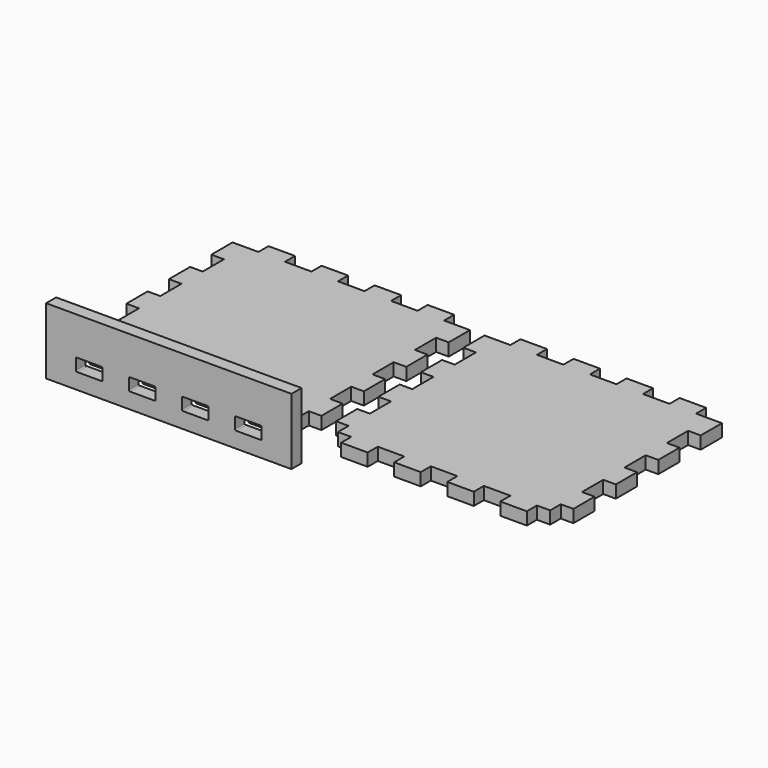
from build123d import *

# Parameters (mm, degrees)
F1_W          = 19
F1_H          = 40
F1_W_2        = 40
F1_H_2        = 19
F2_DEPTH      = 19
F4_W          = 370
F4_H          = 100
F5_DEPTH      = 19
F6_DEPTH      = 188
F7_R          = 1.5
F8_T1_DEPTH   = 17.5
F8_T6_ANGLE   = 233.3892475384
F8_T11_ANGLE  = 233.3892475384
F8_T16_ANGLE  = 233.3892475384
F8_T21_ANGLE  = 233.3892475384
F8_T26_ANGLE  = 233.3892475384
F8_T31_ANGLE  = 233.3892475384
F8_T36_ANGLE  = 233.3892475384
F8_T41_ANGLE  = 233.3892475384
F8_T46_ANGLE  = 233.3892475384
F8_T51_ANGLE  = 233.3892475384
F8_T56_ANGLE  = 233.3892475384
F8_T61_ANGLE  = 233.3892475384
F8_T66_ANGLE  = 233.3892475384
F8_T71_ANGLE  = 233.3892475384
F8_T76_ANGLE  = 233.3892475384
F8_T81_ANGLE  = 233.3892475384
F9_R          = 1.5
F10_T1_DEPTH  = 16
F10_T6_ANGLE  = 233.2969892374
F10_T11_ANGLE = 233.2969892374
F10_T16_ANGLE = 233.2969892374
F10_T21_ANGLE = 233.2969892374
F10_T26_ANGLE = 233.2969892374
F10_T31_ANGLE = 233.2969892374
F10_T36_ANGLE = 233.2969892374
F10_T41_ANGLE = 233.2969892374
F10_T46_ANGLE = 233.2969892374
F10_T51_ANGLE = 233.2969892374
F10_T56_ANGLE = 233.2969892374
F10_T61_ANGLE = 233.2969892374
F10_T66_ANGLE = 233.2969892374
F10_T71_ANGLE = 233.2969892374
F10_T76_ANGLE = 233.2969892374
F10_T81_ANGLE = 233.2969892374
F11_R         = 2.5
F12_DEPTH     = 1


# Not quite as in the source:
# - a fillet or chamfer that OpenCascade refuses, or shapes differently, is made with other operations: its cross-section is extruded or revolved along the edge and cut away or added


with BuildPart() as f2:
    # F1 (on Top) → F2 (new body)
    with BuildSketch(Plane.XY):
        with Locations((15.5, 65)):
            Rectangle(F1_W, F1_H)
        with Locations((15.5, 145)):
            Rectangle(F1_W, F1_H)
        Polygon((25, 85), (25, 45), (25, 25), (45, 25), (85, 25), (125, 25), (165, 25), (205, 25), (245, 25), (285, 25), (325, 25), (345, 25), (345, 45), (345, 85), (345, 125), (345, 165), (345, 205), (345, 245), (345, 285), (345, 325), (325, 325), (285, 325), (245, 325), (205, 325), (165, 325), (125, 325), (85, 325), (45, 325), (25, 325), (25, 285), (25, 245), (25, 205), (25, 165), (25, 125), align=None)
        with Locations((354.5, 65)):
            Rectangle(F1_W, F1_H)
        with Locations((305, 334.5)):
            Rectangle(F1_W_2, F1_H_2)
        with Locations((15.5, 225)):
            Rectangle(F1_W, F1_H)
        with Locations((15.5, 305)):
            Rectangle(F1_W, F1_H)
        with Locations((354.5, 225)):
            Rectangle(F1_W, F1_H)
        with Locations((354.5, 145)):
            Rectangle(F1_W, F1_H)
        with Locations((305, 15.5)):
            Rectangle(F1_W_2, F1_H_2)
        with Locations((225, 15.5)):
            Rectangle(F1_W_2, F1_H_2)
        with Locations((145, 334.5)):
            Rectangle(F1_W_2, F1_H_2)
        with Locations((225, 334.5)):
            Rectangle(F1_W_2, F1_H_2)
        with Locations((145, 15.5)):
            Rectangle(F1_W_2, F1_H_2)
        with Locations((65, 15.5)):
            Rectangle(F1_W_2, F1_H_2)
        with Locations((65, 334.5)):
            Rectangle(F1_W_2, F1_H_2)
        with Locations((354.5, 305)):
            Rectangle(F1_W, F1_H)
    extrude(amount=F2_DEPTH)


with BuildPart() as f3_1:
    # F3: copy of F2
    add(f2.part.moved(Location((380, 0, 0))))


with BuildPart() as f5:
    # F4 (on Front) → F5 (new body)
    with BuildSketch(Plane.XZ):
        with Locations((185, 26.175237447)):
            Rectangle(F4_W, F4_H)
    extrude(amount=F5_DEPTH)

    # F6 (cut): faces of the model
    f6_faces = [f2.part.faces().sort_by_distance(p)[0] for p in [
        (65, 6, 9.5),
        (145, 6, 9.5),
        (225, 6, 9.5),
        (305, 6, 9.5),
    ]]
    extrude(f6_faces, amount=F6_DEPTH, mode=Mode.SUBTRACT)

    # F7
    f7_edges = [f5.edges().sort_by_distance(p)[0] for p in [
        (325, 0, 9.5),
        (285, 0, 9.5),
        (245, 0, 9.5),
        (205, 0, 9.5),
        (165, 0, 9.5),
        (125, 0, 9.5),
        (85, 0, 9.5),
        (45, 0, 9.5),
    ]]
    fillet(f7_edges, radius=F7_R)

    # F8: fillet of radius 1.5 on 16 edges, made by hand

    # F8_s2 → F8_t1 (join)
    with BuildSketch(Plane.XZ.offset(1.5)):
        with BuildLine():
            ThreePointArc((46.5009656854, 19.0004), (45.4393398282, 18.5606601718), (44.9996, 17.4990343146))
            Line((44.9996, 17.4990343146), (44.8494634315, 17.4990343146))
            ThreePointArc((44.8494634315, 17.4990343146), (44.8498634315, 18.2495171573), (44.8498634315, 19))
            Line((44.8498634315, 19), (45, 19.1501365685))
            ThreePointArc((45, 19.1501365685), (45.7504828427, 19.1501365685), (46.5009656854, 19.1505365685))
            Line((46.5009656854, 19.1505365685), (46.5009656854, 19.0004))
        make_face()
        with BuildLine():
            ThreePointArc((46.5009656854, -0.0004), (45.4393398282, 0.4393398282), (44.9996, 1.5009656854))
            Line((44.9996, 1.5009656854), (44.8494634315, 1.5009656854))
            ThreePointArc((44.8494634315, 1.5009656854), (44.8498634315, 0.7504828427), (44.8498634315, 0))
            Line((44.8498634315, 0), (45, -0.1501365685))
            ThreePointArc((45, -0.1501365685), (45.7504828427, -0.1501365685), (46.5009656854, -0.1505365685))
            Line((46.5009656854, -0.1505365685), (46.5009656854, -0.0004))
        make_face()
        with BuildLine():
            ThreePointArc((83.4990343146, 19.0004), (84.5606601718, 18.5606601718), (85.0004, 17.4990343146))
            Line((85.0004, 17.4990343146), (85.1505365685, 17.4990343146))
            ThreePointArc((85.1505365685, 17.4990343146), (85.1501365685, 18.2495171573), (85.1501365685, 19))
            Line((85.1501365685, 19), (85, 19.1501365685))
            ThreePointArc((85, 19.1501365685), (84.2495171573, 19.1501365685), (83.4990343146, 19.1505365685))
            Line((83.4990343146, 19.1505365685), (83.4990343146, 19.0004))
        make_face()
        with BuildLine():
            ThreePointArc((83.4990343146, -0.0004), (84.5606601718, 0.4393398282), (85.0004, 1.5009656854))
            Line((85.0004, 1.5009656854), (85.1505365685, 1.5009656854))
            ThreePointArc((85.1505365685, 1.5009656854), (85.1501365685, 0.7504828427), (85.1501365685, 0))
            Line((85.1501365685, 0), (85, -0.1501365685))
            ThreePointArc((85, -0.1501365685), (84.2495171573, -0.1501365685), (83.4990343146, -0.1505365685))
            Line((83.4990343146, -0.1505365685), (83.4990343146, -0.0004))
        make_face()
        with BuildLine():
            ThreePointArc((126.5009656854, 19.0004), (125.4393398282, 18.5606601718), (124.9996, 17.4990343146))
            Line((124.9996, 17.4990343146), (124.8494634315, 17.4990343146))
            ThreePointArc((124.8494634315, 17.4990343146), (124.8498634315, 18.2495171573), (124.8498634315, 19))
            Line((124.8498634315, 19), (125, 19.1501365685))
            ThreePointArc((125, 19.1501365685), (125.7504828427, 19.1501365685), (126.5009656854, 19.1505365685))
            Line((126.5009656854, 19.1505365685), (126.5009656854, 19.0004))
        make_face()
        with BuildLine():
            ThreePointArc((126.5009656854, -0.0004), (125.4393398282, 0.4393398282), (124.9996, 1.5009656854))
            Line((124.9996, 1.5009656854), (124.8494634315, 1.5009656854))
            ThreePointArc((124.8494634315, 1.5009656854), (124.8498634315, 0.7504828427), (124.8498634315, 0))
            Line((124.8498634315, 0), (125, -0.1501365685))
            ThreePointArc((125, -0.1501365685), (125.7504828427, -0.1501365685), (126.5009656854, -0.1505365685))
            Line((126.5009656854, -0.1505365685), (126.5009656854, -0.0004))
        make_face()
        with BuildLine():
            ThreePointArc((163.4990343146, -0.0004), (164.5606601718, 0.4393398282), (165.0004, 1.5009656854))
            Line((165.0004, 1.5009656854), (165.1505365685, 1.5009656854))
            ThreePointArc((165.1505365685, 1.5009656854), (165.1501365685, 0.7504828427), (165.1501365685, 0))
            Line((165.1501365685, 0), (165, -0.1501365685))
            ThreePointArc((165, -0.1501365685), (164.2495171573, -0.1501365685), (163.4990343146, -0.1505365685))
            Line((163.4990343146, -0.1505365685), (163.4990343146, -0.0004))
        make_face()
        with BuildLine():
            ThreePointArc((206.5009656854, -0.0004), (205.4393398282, 0.4393398282), (204.9996, 1.5009656854))
            Line((204.9996, 1.5009656854), (204.8494634315, 1.5009656854))
            ThreePointArc((204.8494634315, 1.5009656854), (204.8498634315, 0.7504828427), (204.8498634315, 0))
            Line((204.8498634315, 0), (205, -0.1501365685))
            ThreePointArc((205, -0.1501365685), (205.7504828427, -0.1501365685), (206.5009656854, -0.1505365685))
            Line((206.5009656854, -0.1505365685), (206.5009656854, -0.0004))
        make_face()
        with BuildLine():
            ThreePointArc((206.5009656854, 19.0004), (205.4393398282, 18.5606601718), (204.9996, 17.4990343146))
            Line((204.9996, 17.4990343146), (204.8494634315, 17.4990343146))
            ThreePointArc((204.8494634315, 17.4990343146), (204.8498634315, 18.2495171573), (204.8498634315, 19))
            Line((204.8498634315, 19), (205, 19.1501365685))
            ThreePointArc((205, 19.1501365685), (205.7504828427, 19.1501365685), (206.5009656854, 19.1505365685))
            Line((206.5009656854, 19.1505365685), (206.5009656854, 19.0004))
        make_face()
        with BuildLine():
            ThreePointArc((243.4990343146, -0.0004), (244.5606601718, 0.4393398282), (245.0004, 1.5009656854))
            Line((245.0004, 1.5009656854), (245.1505365685, 1.5009656854))
            ThreePointArc((245.1505365685, 1.5009656854), (245.1501365685, 0.7504828427), (245.1501365685, 0))
            Line((245.1501365685, 0), (245, -0.1501365685))
            ThreePointArc((245, -0.1501365685), (244.2495171573, -0.1501365685), (243.4990343146, -0.1505365685))
            Line((243.4990343146, -0.1505365685), (243.4990343146, -0.0004))
        make_face()
        with BuildLine():
            ThreePointArc((243.4990343146, 19.0004), (244.5606601718, 18.5606601718), (245.0004, 17.4990343146))
            Line((245.0004, 17.4990343146), (245.1505365685, 17.4990343146))
            ThreePointArc((245.1505365685, 17.4990343146), (245.1501365685, 18.2495171573), (245.1501365685, 19))
            Line((245.1501365685, 19), (245, 19.1501365685))
            ThreePointArc((245, 19.1501365685), (244.2495171573, 19.1501365685), (243.4990343146, 19.1505365685))
            Line((243.4990343146, 19.1505365685), (243.4990343146, 19.0004))
        make_face()
        with BuildLine():
            ThreePointArc((323.4990343146, 19.0004), (324.5606601718, 18.5606601718), (325.0004, 17.4990343146))
            Line((325.0004, 17.4990343146), (325.1505365685, 17.4990343146))
            ThreePointArc((325.1505365685, 17.4990343146), (325.1501365685, 18.2495171573), (325.1501365685, 19))
            Line((325.1501365685, 19), (325, 19.1501365685))
            ThreePointArc((325, 19.1501365685), (324.2495171573, 19.1501365685), (323.4990343146, 19.1505365685))
            Line((323.4990343146, 19.1505365685), (323.4990343146, 19.0004))
        make_face()
        with BuildLine():
            ThreePointArc((286.5009656854, 19.0004), (285.4393398282, 18.5606601718), (284.9996, 17.4990343146))
            Line((284.9996, 17.4990343146), (284.8494634315, 17.4990343146))
            ThreePointArc((284.8494634315, 17.4990343146), (284.8498634315, 18.2495171573), (284.8498634315, 19))
            Line((284.8498634315, 19), (285, 19.1501365685))
            ThreePointArc((285, 19.1501365685), (285.7504828427, 19.1501365685), (286.5009656854, 19.1505365685))
            Line((286.5009656854, 19.1505365685), (286.5009656854, 19.0004))
        make_face()
        with BuildLine():
            ThreePointArc((163.4990343146, 19.0004), (164.5606601718, 18.5606601718), (165.0004, 17.4990343146))
            Line((165.0004, 17.4990343146), (165.1505365685, 17.4990343146))
            ThreePointArc((165.1505365685, 17.4990343146), (165.1501365685, 18.2495171573), (165.1501365685, 19))
            Line((165.1501365685, 19), (165, 19.1501365685))
            ThreePointArc((165, 19.1501365685), (164.2495171573, 19.1501365685), (163.4990343146, 19.1505365685))
            Line((163.4990343146, 19.1505365685), (163.4990343146, 19.0004))
        make_face()
        with BuildLine():
            ThreePointArc((286.5009656854, -0.0004), (285.4393398282, 0.4393398282), (284.9996, 1.5009656854))
            Line((284.9996, 1.5009656854), (284.8494634315, 1.5009656854))
            ThreePointArc((284.8494634315, 1.5009656854), (284.8498634315, 0.7504828427), (284.8498634315, 0))
            Line((284.8498634315, 0), (285, -0.1501365685))
            ThreePointArc((285, -0.1501365685), (285.7504828427, -0.1501365685), (286.5009656854, -0.1505365685))
            Line((286.5009656854, -0.1505365685), (286.5009656854, -0.0004))
        make_face()
        with BuildLine():
            ThreePointArc((323.4990343146, -0.0004), (324.5606601718, 0.4393398282), (325.0004, 1.5009656854))
            Line((325.0004, 1.5009656854), (325.1505365685, 1.5009656854))
            ThreePointArc((325.1505365685, 1.5009656854), (325.1501365685, 0.7504828427), (325.1501365685, 0))
            Line((325.1501365685, 0), (325, -0.1501365685))
            ThreePointArc((325, -0.1501365685), (324.2495171573, -0.1501365685), (323.4990343146, -0.1505365685))
            Line((323.4990343146, -0.1505365685), (323.4990343146, -0.0004))
        make_face()
    extrude(amount=F8_T1_DEPTH)


with BuildPart() as f8_tool4:
    # F8_s5 → F8_t6 (revolve)
    with BuildSketch(Plane(origin=(209.6577088502, 155.7666111289, 0), x_dir=(0, 0, 1), z_dir=(-0.80270557, -0.5963755259, 0))):
        with BuildLine():
            ThreePointArc((1.5009656854, -197.4202675598), (0.4393398282, -197.8600073881), (-0.0004, -198.9216332453))
            Line((-0.0004, -198.9216332453), (-0.1505365685, -198.9216332453))
            ThreePointArc((-0.1505365685, -198.9216332453), (-0.1501365685, -198.1711504026), (-0.1501365685, -197.4206675598))
            Line((-0.1501365685, -197.4206675598), (0, -197.2705309913))
            ThreePointArc((0, -197.2705309913), (0.7504828427, -197.2705309913), (1.5009656854, -197.2701309913))
            Line((1.5009656854, -197.2701309913), (1.5009656854, -197.4202675598))
        make_face()
    revolve(axis=Axis((326.5, -1.5, 0), (0, 0, 1)), revolution_arc=F8_T6_ANGLE)

    split(bisect_by=Plane.XZ, keep=Keep.TOP)


with BuildPart() as f5_1:
    add(f5.part)

    # F8_t3: union F8_tool4
    add(f8_tool4.part)


with BuildPart() as f8_tool9:
    # F8_s10 → F8_t11 (revolve)
    with BuildSketch(Plane(origin=(183.3873927387, -136.2489023052, 0), x_dir=(0, 0, 1), z_dir=(0.80270557, -0.5963755259, 0))):
        with BuildLine():
            ThreePointArc((-0.0004, -164.8674375509), (0.4393398282, -165.9290634081), (1.5009656854, -166.3688032363))
            Line((1.5009656854, -166.3688032363), (1.5009656854, -166.5189398049))
            ThreePointArc((1.5009656854, -166.5189398049), (0.7504828427, -166.5185398049), (0, -166.5185398049))
            Line((0, -166.5185398049), (-0.1501365685, -166.3684032363))
            ThreePointArc((-0.1501365685, -166.3684032363), (-0.1501365685, -165.6179203936), (-0.1505365685, -164.8674375509))
            Line((-0.1505365685, -164.8674375509), (-0.0004, -164.8674375509))
        make_face()
    revolve(axis=Axis((283.5, -1.5, 0), (0, 0, -1)), revolution_arc=F8_T11_ANGLE)

    split(bisect_by=Plane.XZ, keep=Keep.TOP)


with BuildPart() as f5_2:
    add(f5_1.part)

    # F8_t8: union F8_tool9
    add(f8_tool9.part)


with BuildPart() as f8_tool14:
    # F8_s15 → F8_t16 (revolve)
    with BuildSketch(Plane(origin=(106.5639117121, 79.172378097, 0), x_dir=(0, 0, 1), z_dir=(-0.80270557, -0.5963755259, 0))):
        with BuildLine():
            ThreePointArc((19.0004, -103.501549102), (18.5606601718, -102.4399232448), (17.4990343146, -102.0001834166))
            Line((17.4990343146, -102.0001834166), (17.4990343146, -101.850046848))
            ThreePointArc((17.4990343146, -101.850046848), (18.2495171573, -101.850446848), (19, -101.850446848))
            Line((19, -101.850446848), (19.1501365685, -102.0005834166))
            ThreePointArc((19.1501365685, -102.0005834166), (19.1501365685, -102.7510662593), (19.1505365685, -103.501549102))
            Line((19.1505365685, -103.501549102), (19.0004, -103.501549102))
        make_face()
    revolve(axis=Axis((166.5, -1.5, 19), (0, 0, 1)), revolution_arc=F8_T16_ANGLE)

    split(bisect_by=Plane.XZ, keep=Keep.TOP)


with BuildPart() as f5_3:
    add(f5_2.part)

    # F8_t13: union F8_tool14
    add(f8_tool14.part)


with BuildPart() as f8_tool19:
    # F8_s20 → F8_t21 (revolve)
    with BuildSketch(Plane(origin=(183.3873927387, -136.2489023052, 0), x_dir=(0, 0, 1), z_dir=(0.80270557, -0.5963755259, 0))):
        with BuildLine():
            ThreePointArc((19.0004, -164.8674375509), (18.5606601718, -165.9290634081), (17.4990343146, -166.3688032363))
            Line((17.4990343146, -166.3688032363), (17.4990343146, -166.5189398049))
            ThreePointArc((17.4990343146, -166.5189398049), (18.2495171573, -166.5185398049), (19, -166.5185398049))
            Line((19, -166.5185398049), (19.1501365685, -166.3684032363))
            ThreePointArc((19.1501365685, -166.3684032363), (19.1501365685, -165.6179203936), (19.1505365685, -164.8674375509))
            Line((19.1505365685, -164.8674375509), (19.0004, -164.8674375509))
        make_face()
    revolve(axis=Axis((283.5, -1.5, 19), (0, 0, -1)), revolution_arc=F8_T21_ANGLE)

    split(bisect_by=Plane.XZ, keep=Keep.TOP)


with BuildPart() as f5_4:
    add(f5_3.part)

    # F8_t18: union F8_tool19
    add(f8_tool19.part)


with BuildPart() as f8_tool24:
    # F8_s25 → F8_t26 (revolve)
    with BuildSketch(Plane(origin=(209.6577088502, 155.7666111289, 0), x_dir=(0, 0, 1), z_dir=(-0.80270557, -0.5963755259, 0))):
        with BuildLine():
            ThreePointArc((19.0004, -198.9216332453), (18.5606601718, -197.8600073881), (17.4990343146, -197.4202675598))
            Line((17.4990343146, -197.4202675598), (17.4990343146, -197.2701309913))
            ThreePointArc((17.4990343146, -197.2701309913), (18.2495171573, -197.2705309913), (19, -197.2705309913))
            Line((19, -197.2705309913), (19.1501365685, -197.4206675598))
            ThreePointArc((19.1501365685, -197.4206675598), (19.1501365685, -198.1711504026), (19.1505365685, -198.9216332453))
            Line((19.1505365685, -198.9216332453), (19.0004, -198.9216332453))
        make_face()
    revolve(axis=Axis((326.5, -1.5, 19), (0, 0, 1)), revolution_arc=F8_T26_ANGLE)

    split(bisect_by=Plane.XZ, keep=Keep.TOP)


with BuildPart() as f5_5:
    add(f5_4.part)

    # F8_t23: union F8_tool24
    add(f8_tool24.part)


with BuildPart() as f8_tool29:
    # F8_s30 → F8_t31 (revolve)
    with BuildSketch(Plane(origin=(158.1108102812, 117.4694946129, 0), x_dir=(0, 0, 1), z_dir=(-0.80270557, -0.5963755259, 0))):
        with BuildLine():
            ThreePointArc((19.0004, -151.2115911736), (18.5606601718, -150.1499653164), (17.4990343146, -149.7102254882))
            Line((17.4990343146, -149.7102254882), (17.4990343146, -149.5600889197))
            ThreePointArc((17.4990343146, -149.5600889197), (18.2495171573, -149.5604889197), (19, -149.5604889197))
            Line((19, -149.5604889197), (19.1501365685, -149.7106254882))
            ThreePointArc((19.1501365685, -149.7106254882), (19.1501365685, -150.4611083309), (19.1505365685, -151.2115911736))
            Line((19.1505365685, -151.2115911736), (19.0004, -151.2115911736))
        make_face()
    revolve(axis=Axis((246.5, -1.5, 19), (0, 0, 1)), revolution_arc=F8_T31_ANGLE)

    split(bisect_by=Plane.XZ, keep=Keep.TOP)


with BuildPart() as f5_6:
    add(f5_5.part)

    # F8_t28: union F8_tool29
    add(f8_tool29.part)


with BuildPart() as f8_tool34:
    # F8_s35 → F8_t36 (revolve)
    with BuildSketch(Plane(origin=(158.1108102812, 117.4694946129, 0), x_dir=(0, 0, 1), z_dir=(-0.80270557, -0.5963755259, 0))):
        with BuildLine():
            ThreePointArc((1.5009656854, -149.7102254882), (0.4393398282, -150.1499653164), (-0.0004, -151.2115911736))
            Line((-0.0004, -151.2115911736), (-0.1505365685, -151.2115911736))
            ThreePointArc((-0.1505365685, -151.2115911736), (-0.1501365685, -150.4611083309), (-0.1501365685, -149.7106254882))
            Line((-0.1501365685, -149.7106254882), (0, -149.5604889197))
            ThreePointArc((0, -149.5604889197), (0.7504828427, -149.5604889197), (1.5009656854, -149.5600889197))
            Line((1.5009656854, -149.5600889197), (1.5009656854, -149.7102254882))
        make_face()
    revolve(axis=Axis((246.5, -1.5, 0), (0, 0, 1)), revolution_arc=F8_T36_ANGLE)

    split(bisect_by=Plane.XZ, keep=Keep.TOP)


with BuildPart() as f5_7:
    add(f5_6.part)

    # F8_t33: union F8_tool34
    add(f8_tool34.part)


with BuildPart() as f8_tool39:
    # F8_s40 → F8_t41 (revolve)
    with BuildSketch(Plane(origin=(131.8404941697, -97.9517857893, 0), x_dir=(0, 0, 1), z_dir=(0.80270557, -0.5963755259, 0))):
        with BuildLine():
            ThreePointArc((19.0004, -117.1573954793), (18.5606601718, -118.2190213365), (17.4990343146, -118.6587611647))
            Line((17.4990343146, -118.6587611647), (17.4990343146, -118.8088977333))
            ThreePointArc((17.4990343146, -118.8088977333), (18.2495171573, -118.8084977333), (19, -118.8084977333))
            Line((19, -118.8084977333), (19.1501365685, -118.6583611647))
            ThreePointArc((19.1501365685, -118.6583611647), (19.1501365685, -117.907878322), (19.1505365685, -117.1573954793))
            Line((19.1505365685, -117.1573954793), (19.0004, -117.1573954793))
        make_face()
    revolve(axis=Axis((203.5, -1.5, 19), (0, 0, -1)), revolution_arc=F8_T41_ANGLE)

    split(bisect_by=Plane.XZ, keep=Keep.TOP)


with BuildPart() as f5_8:
    add(f5_7.part)

    # F8_t38: union F8_tool39
    add(f8_tool39.part)


with BuildPart() as f8_tool44:
    # F8_s45 → F8_t46 (revolve)
    with BuildSketch(Plane(origin=(131.8404941697, -97.9517857893, 0), x_dir=(0, 0, 1), z_dir=(0.80270557, -0.5963755259, 0))):
        with BuildLine():
            ThreePointArc((-0.0004, -117.1573954793), (0.4393398282, -118.2190213365), (1.5009656854, -118.6587611647))
            Line((1.5009656854, -118.6587611647), (1.5009656854, -118.8088977333))
            ThreePointArc((1.5009656854, -118.8088977333), (0.7504828427, -118.8084977333), (0, -118.8084977333))
            Line((0, -118.8084977333), (-0.1501365685, -118.6583611647))
            ThreePointArc((-0.1501365685, -118.6583611647), (-0.1501365685, -117.907878322), (-0.1505365685, -117.1573954793))
            Line((-0.1505365685, -117.1573954793), (-0.0004, -117.1573954793))
        make_face()
    revolve(axis=Axis((203.5, -1.5, 0), (0, 0, -1)), revolution_arc=F8_T46_ANGLE)

    split(bisect_by=Plane.XZ, keep=Keep.TOP)


with BuildPart() as f5_9:
    add(f5_8.part)

    # F8_t43: union F8_tool44
    add(f8_tool44.part)


with BuildPart() as f8_tool49:
    # F8_s50 → F8_t51 (revolve)
    with BuildSketch(Plane(origin=(106.5639117121, 79.172378097, 0), x_dir=(0, 0, 1), z_dir=(-0.80270557, -0.5963755259, 0))):
        with BuildLine():
            ThreePointArc((1.5009656854, -102.0001834166), (0.4393398282, -102.4399232448), (-0.0004, -103.501549102))
            Line((-0.0004, -103.501549102), (-0.1505365685, -103.501549102))
            ThreePointArc((-0.1505365685, -103.501549102), (-0.1501365685, -102.7510662593), (-0.1501365685, -102.0005834166))
            Line((-0.1501365685, -102.0005834166), (0, -101.850446848))
            ThreePointArc((0, -101.850446848), (0.7504828427, -101.850446848), (1.5009656854, -101.850046848))
            Line((1.5009656854, -101.850046848), (1.5009656854, -102.0001834166))
        make_face()
    revolve(axis=Axis((166.5, -1.5, 0), (0, 0, 1)), revolution_arc=F8_T51_ANGLE)

    split(bisect_by=Plane.XZ, keep=Keep.TOP)


with BuildPart() as f5_10:
    add(f5_9.part)

    # F8_t48: union F8_tool49
    add(f8_tool49.part)


with BuildPart() as f8_tool54:
    # F8_s55 → F8_t56 (revolve)
    with BuildSketch(Plane(origin=(80.2935956006, -59.6546692733, 0), x_dir=(0, 0, 1), z_dir=(0.80270557, -0.5963755259, 0))):
        with BuildLine():
            ThreePointArc((-0.0004, -69.4473534077), (0.4393398282, -70.5089792649), (1.5009656854, -70.9487190931))
            Line((1.5009656854, -70.9487190931), (1.5009656854, -71.0988556616))
            ThreePointArc((1.5009656854, -71.0988556616), (0.7504828427, -71.0984556616), (0, -71.0984556616))
            Line((0, -71.0984556616), (-0.1501365685, -70.9483190931))
            ThreePointArc((-0.1501365685, -70.9483190931), (-0.1501365685, -70.1978362504), (-0.1505365685, -69.4473534077))
            Line((-0.1505365685, -69.4473534077), (-0.0004, -69.4473534077))
        make_face()
    revolve(axis=Axis((123.5, -1.5, 0), (0, 0, -1)), revolution_arc=F8_T56_ANGLE)

    split(bisect_by=Plane.XZ, keep=Keep.TOP)


with BuildPart() as f5_11:
    add(f5_10.part)

    # F8_t53: union F8_tool54
    add(f8_tool54.part)


with BuildPart() as f8_tool59:
    # F8_s60 → F8_t61 (revolve)
    with BuildSketch(Plane(origin=(80.2935956006, -59.6546692733, 0), x_dir=(0, 0, 1), z_dir=(0.80270557, -0.5963755259, 0))):
        with BuildLine():
            ThreePointArc((19.0004, -69.4473534077), (18.5606601718, -70.5089792649), (17.4990343146, -70.9487190931))
            Line((17.4990343146, -70.9487190931), (17.4990343146, -71.0988556616))
            ThreePointArc((17.4990343146, -71.0988556616), (18.2495171573, -71.0984556616), (19, -71.0984556616))
            Line((19, -71.0984556616), (19.1501365685, -70.9483190931))
            ThreePointArc((19.1501365685, -70.9483190931), (19.1501365685, -70.1978362504), (19.1505365685, -69.4473534077))
            Line((19.1505365685, -69.4473534077), (19.0004, -69.4473534077))
        make_face()
    revolve(axis=Axis((123.5, -1.5, 19), (0, 0, -1)), revolution_arc=F8_T61_ANGLE)

    split(bisect_by=Plane.XZ, keep=Keep.TOP)


with BuildPart() as f5_12:
    add(f5_11.part)

    # F8_t58: union F8_tool59
    add(f8_tool59.part)


with BuildPart() as f8_tool64:
    # F8_s65 → F8_t66 (revolve)
    with BuildSketch(Plane(origin=(55.0170131431, 40.875261581, 0), x_dir=(0, 0, 1), z_dir=(-0.80270557, -0.5963755259, 0))):
        with BuildLine():
            ThreePointArc((1.5009656854, -54.290141345), (0.4393398282, -54.7298811732), (-0.0004, -55.7915070304))
            Line((-0.0004, -55.7915070304), (-0.1505365685, -55.7915070304))
            ThreePointArc((-0.1505365685, -55.7915070304), (-0.1501365685, -55.0410241877), (-0.1501365685, -54.290541345))
            Line((-0.1501365685, -54.290541345), (0, -54.1404047764))
            ThreePointArc((0, -54.1404047764), (0.7504828427, -54.1404047764), (1.5009656854, -54.1400047764))
            Line((1.5009656854, -54.1400047764), (1.5009656854, -54.290141345))
        make_face()
    revolve(axis=Axis((86.5, -1.5, 0), (0, 0, 1)), revolution_arc=F8_T66_ANGLE)

    split(bisect_by=Plane.XZ, keep=Keep.TOP)


with BuildPart() as f5_13:
    add(f5_12.part)

    # F8_t63: union F8_tool64
    add(f8_tool64.part)


with BuildPart() as f8_tool69:
    # F8_s70 → F8_t71 (revolve)
    with BuildSketch(Plane(origin=(55.0170131431, 40.875261581, 0), x_dir=(0, 0, 1), z_dir=(-0.80270557, -0.5963755259, 0))):
        with BuildLine():
            ThreePointArc((19.0004, -55.7915070304), (18.5606601718, -54.7298811732), (17.4990343146, -54.290141345))
            Line((17.4990343146, -54.290141345), (17.4990343146, -54.1400047764))
            ThreePointArc((17.4990343146, -54.1400047764), (18.2495171573, -54.1404047764), (19, -54.1404047764))
            Line((19, -54.1404047764), (19.1501365685, -54.290541345))
            ThreePointArc((19.1501365685, -54.290541345), (19.1501365685, -55.0410241877), (19.1505365685, -55.7915070304))
            Line((19.1505365685, -55.7915070304), (19.0004, -55.7915070304))
        make_face()
    revolve(axis=Axis((86.5, -1.5, 19), (0, 0, 1)), revolution_arc=F8_T71_ANGLE)

    split(bisect_by=Plane.XZ, keep=Keep.TOP)


with BuildPart() as f5_14:
    add(f5_13.part)

    # F8_t68: union F8_tool69
    add(f8_tool69.part)


with BuildPart() as f8_tool74:
    # F8_s75 → F8_t76 (revolve)
    with BuildSketch(Plane(origin=(28.7466970316, -21.3575527574, 0), x_dir=(0, 0, 1), z_dir=(0.80270557, -0.5963755259, 0))):
        with BuildLine():
            ThreePointArc((-0.0004, -21.737311336), (0.4393398282, -22.7989371932), (1.5009656854, -23.2386770214))
            Line((1.5009656854, -23.2386770214), (1.5009656854, -23.38881359))
            ThreePointArc((1.5009656854, -23.38881359), (0.7504828427, -23.38841359), (0, -23.38841359))
            Line((0, -23.38841359), (-0.1501365685, -23.2382770214))
            ThreePointArc((-0.1501365685, -23.2382770214), (-0.1501365685, -22.4877941787), (-0.1505365685, -21.737311336))
            Line((-0.1505365685, -21.737311336), (-0.0004, -21.737311336))
        make_face()
    revolve(axis=Axis((43.5, -1.5, 0), (0, 0, -1)), revolution_arc=F8_T76_ANGLE)

    split(bisect_by=Plane.XZ, keep=Keep.TOP)


with BuildPart() as f5_15:
    add(f5_14.part)

    # F8_t73: union F8_tool74
    add(f8_tool74.part)


with BuildPart() as f8_tool79:
    # F8_s80 → F8_t81 (revolve)
    with BuildSketch(Plane(origin=(28.7466970316, -21.3575527574, 0), x_dir=(0, 0, 1), z_dir=(0.80270557, -0.5963755259, 0))):
        with BuildLine():
            ThreePointArc((19.0004, -21.737311336), (18.5606601718, -22.7989371932), (17.4990343146, -23.2386770214))
            Line((17.4990343146, -23.2386770214), (17.4990343146, -23.38881359))
            ThreePointArc((17.4990343146, -23.38881359), (18.2495171573, -23.38841359), (19, -23.38841359))
            Line((19, -23.38841359), (19.1501365685, -23.2382770214))
            ThreePointArc((19.1501365685, -23.2382770214), (19.1501365685, -22.4877941787), (19.1505365685, -21.737311336))
            Line((19.1505365685, -21.737311336), (19.0004, -21.737311336))
        make_face()
    revolve(axis=Axis((43.5, -1.5, 19), (0, 0, -1)), revolution_arc=F8_T81_ANGLE)

    split(bisect_by=Plane.XZ, keep=Keep.TOP)


with BuildPart() as f5_16:
    add(f5_15.part)

    # F8_t78: union F8_tool79
    add(f8_tool79.part)

    # F11 (on face) → F12 (cut)
    with BuildSketch(Plane(origin=(0, 0, 0), x_dir=(-1, 0, 0), z_dir=(0, 1, 0))):
        with Locations((-10, 66.175237447)):
            Circle(F11_R)
    extrude(amount=-F12_DEPTH, mode=Mode.SUBTRACT)


with BuildPart() as f2_1:
    add(f2.part)

    # F9
    f9_edges = [f2_1.edges().sort_by_distance(p)[0] for p in [
        (45, 15.5, 19),
        (85, 15.5, 19),
        (125, 15.5, 19),
        (165, 15.5, 19),
        (205, 15.5, 19),
        (245, 15.5, 19),
        (285, 15.5, 19),
        (325, 15.5, 19),
        (45, 15.5, 0),
        (85, 15.5, 0),
        (125, 15.5, 0),
        (165, 15.5, 0),
        (205, 15.5, 0),
        (245, 15.5, 0),
        (285, 15.5, 0),
        (325, 15.5, 0),
    ]]
    fillet(f9_edges, radius=F9_R)

    # F10: fillet of radius 1.5 on 8 edges, made by hand

    # F10_s2 → F10_t1 (join)
    with BuildSketch(Plane.XY.offset(1.5)):
        with BuildLine():
            ThreePointArc((86.5, 25), (85.4393398282, 24.5606601718), (85, 23.5))
            Line((85, 23.5), (85, 25))
            Line((85, 25), (86.5, 25))
        make_face()
        with BuildLine():
            ThreePointArc((166.5, 25), (165.4393398282, 24.5606601718), (165, 23.5))
            Line((165, 23.5), (165, 25))
            Line((165, 25), (166.5, 25))
        make_face()
        with BuildLine():
            ThreePointArc((246.5, 25), (245.4393398282, 24.5606601718), (245, 23.5))
            Line((245, 23.5), (245, 25))
            Line((245, 25), (246.5, 25))
        make_face()
        with BuildLine():
            ThreePointArc((326.5, 25), (325.4393398282, 24.5606601718), (325, 23.5))
            Line((325, 23.5), (325, 25))
            Line((325, 25), (326.5, 25))
        make_face()
        with BuildLine():
            ThreePointArc((283.5, 25), (284.5606601718, 24.5606601718), (285, 23.5))
            Line((285, 23.5), (285, 25))
            Line((285, 25), (283.5, 25))
        make_face()
        with BuildLine():
            ThreePointArc((203.5, 25), (204.5606601718, 24.5606601718), (205, 23.5))
            Line((205, 23.5), (205, 25))
            Line((205, 25), (203.5, 25))
        make_face()
        with BuildLine():
            ThreePointArc((123.5, 25), (124.5606601718, 24.5606601718), (125, 23.5))
            Line((125, 23.5), (125, 25))
            Line((125, 25), (123.5, 25))
        make_face()
        with BuildLine():
            ThreePointArc((43.5, 25), (44.5606601718, 24.5606601718), (45, 23.5))
            Line((45, 23.5), (45, 25))
            Line((45, 25), (43.5, 25))
        make_face()
    extrude(amount=F10_T1_DEPTH)


with BuildPart() as f10_tool4:
    # F10_s5 → F10_t6 (revolve)
    with BuildSketch(Plane.XY.offset(1.5)):
        with BuildLine():
            ThreePointArc((43.5, 25), (44.5606601718, 24.5606601718), (45, 23.5))
            Line((45, 23.5), (45, 25))
            Line((45, 25), (43.5, 25))
        make_face()
    revolve(axis=Axis((46.5, 25, 1.5), (0, -1, 0)), revolution_arc=F10_T6_ANGLE)

    split(bisect_by=Plane.XY, keep=Keep.TOP)


with BuildPart() as f2_2:
    add(f2_1.part)

    # F10_t3: union F10_tool4
    add(f10_tool4.part)


with BuildPart() as f10_tool9:
    # F10_s10 → F10_t11 (revolve)
    with BuildSketch(Plane.XY.offset(17.5)):
        with BuildLine():
            ThreePointArc((43.5, 25), (44.5606601718, 24.5606601718), (45, 23.5))
            Line((45, 23.5), (45, 25))
            Line((45, 25), (43.5, 25))
        make_face()
    revolve(axis=Axis((46.5, 25, 17.5), (0, 1, 0)), revolution_arc=F10_T11_ANGLE)

    split(bisect_by=Plane.XY.offset(19), keep=Keep.BOTTOM)


with BuildPart() as f2_3:
    add(f2_2.part)

    # F10_t8: union F10_tool9
    add(f10_tool9.part)


with BuildPart() as f10_tool14:
    # F10_s15 → F10_t16 (revolve)
    with BuildSketch(Plane.XY.offset(1.5)):
        with BuildLine():
            ThreePointArc((123.5, 25), (124.5606601718, 24.5606601718), (125, 23.5))
            Line((125, 23.5), (125, 25))
            Line((125, 25), (123.5, 25))
        make_face()
    revolve(axis=Axis((126.5, 25, 1.5), (0, -1, 0)), revolution_arc=F10_T16_ANGLE)

    split(bisect_by=Plane.XY, keep=Keep.TOP)


with BuildPart() as f2_4:
    add(f2_3.part)

    # F10_t13: union F10_tool14
    add(f10_tool14.part)


with BuildPart() as f10_tool19:
    # F10_s20 → F10_t21 (revolve)
    with BuildSketch(Plane.XY.offset(17.5)):
        with BuildLine():
            ThreePointArc((123.5, 25), (124.5606601718, 24.5606601718), (125, 23.5))
            Line((125, 23.5), (125, 25))
            Line((125, 25), (123.5, 25))
        make_face()
    revolve(axis=Axis((126.5, 25, 17.5), (0, 1, 0)), revolution_arc=F10_T21_ANGLE)

    split(bisect_by=Plane.XY.offset(19), keep=Keep.BOTTOM)


with BuildPart() as f2_5:
    add(f2_4.part)

    # F10_t18: union F10_tool19
    add(f10_tool19.part)


with BuildPart() as f10_tool24:
    # F10_s25 → F10_t26 (revolve)
    with BuildSketch(Plane.XY.offset(1.5)):
        with BuildLine():
            ThreePointArc((203.5, 25), (204.5606601718, 24.5606601718), (205, 23.5))
            Line((205, 23.5), (205, 25))
            Line((205, 25), (203.5, 25))
        make_face()
    revolve(axis=Axis((206.5, 25, 1.5), (0, -1, 0)), revolution_arc=F10_T26_ANGLE)

    split(bisect_by=Plane.XY, keep=Keep.TOP)


with BuildPart() as f2_6:
    add(f2_5.part)

    # F10_t23: union F10_tool24
    add(f10_tool24.part)


with BuildPart() as f10_tool29:
    # F10_s30 → F10_t31 (revolve)
    with BuildSketch(Plane.XY.offset(17.5)):
        with BuildLine():
            ThreePointArc((203.5, 25), (204.5606601718, 24.5606601718), (205, 23.5))
            Line((205, 23.5), (205, 25))
            Line((205, 25), (203.5, 25))
        make_face()
    revolve(axis=Axis((206.5, 25, 17.5), (0, 1, 0)), revolution_arc=F10_T31_ANGLE)

    split(bisect_by=Plane.XY.offset(19), keep=Keep.BOTTOM)


with BuildPart() as f2_7:
    add(f2_6.part)

    # F10_t28: union F10_tool29
    add(f10_tool29.part)


with BuildPart() as f10_tool34:
    # F10_s35 → F10_t36 (revolve)
    with BuildSketch(Plane.XY.offset(1.5)):
        with BuildLine():
            ThreePointArc((283.5, 25), (284.5606601718, 24.5606601718), (285, 23.5))
            Line((285, 23.5), (285, 25))
            Line((285, 25), (283.5, 25))
        make_face()
    revolve(axis=Axis((286.5, 25, 1.5), (0, -1, 0)), revolution_arc=F10_T36_ANGLE)

    split(bisect_by=Plane.XY, keep=Keep.TOP)


with BuildPart() as f2_8:
    add(f2_7.part)

    # F10_t33: union F10_tool34
    add(f10_tool34.part)


with BuildPart() as f10_tool39:
    # F10_s40 → F10_t41 (revolve)
    with BuildSketch(Plane.XY.offset(17.5)):
        with BuildLine():
            ThreePointArc((283.5, 25), (284.5606601718, 24.5606601718), (285, 23.5))
            Line((285, 23.5), (285, 25))
            Line((285, 25), (283.5, 25))
        make_face()
    revolve(axis=Axis((286.5, 25, 17.5), (0, 1, 0)), revolution_arc=F10_T41_ANGLE)

    split(bisect_by=Plane.XY.offset(19), keep=Keep.BOTTOM)


with BuildPart() as f2_9:
    add(f2_8.part)

    # F10_t38: union F10_tool39
    add(f10_tool39.part)


with BuildPart() as f10_tool44:
    # F10_s45 → F10_t46 (revolve)
    with BuildSketch(Plane.XY.offset(1.5)):
        with BuildLine():
            ThreePointArc((325, 23.5), (325.4393398282, 24.5606601718), (326.5, 25))
            Line((326.5, 25), (325, 25))
            Line((325, 25), (325, 23.5))
        make_face()
    revolve(axis=Axis((323.5, 25, 1.5), (0, 1, 0)), revolution_arc=F10_T46_ANGLE)

    split(bisect_by=Plane.XY, keep=Keep.TOP)


with BuildPart() as f2_10:
    add(f2_9.part)

    # F10_t43: union F10_tool44
    add(f10_tool44.part)


with BuildPart() as f10_tool49:
    # F10_s50 → F10_t51 (revolve)
    with BuildSketch(Plane.XY.offset(17.5)):
        with BuildLine():
            ThreePointArc((326.5, 25), (325.4393398282, 24.5606601718), (325, 23.5))
            Line((325, 23.5), (325, 25))
            Line((325, 25), (326.5, 25))
        make_face()
    revolve(axis=Axis((323.5, 25, 17.5), (0, -1, 0)), revolution_arc=F10_T51_ANGLE)

    split(bisect_by=Plane.XY.offset(19), keep=Keep.BOTTOM)


with BuildPart() as f2_11:
    add(f2_10.part)

    # F10_t48: union F10_tool49
    add(f10_tool49.part)


with BuildPart() as f10_tool54:
    # F10_s55 → F10_t56 (revolve)
    with BuildSketch(Plane.XY.offset(1.5)):
        with BuildLine():
            ThreePointArc((245, 23.5), (245.4393398282, 24.5606601718), (246.5, 25))
            Line((246.5, 25), (245, 25))
            Line((245, 25), (245, 23.5))
        make_face()
    revolve(axis=Axis((243.5, 25, 1.5), (0, 1, 0)), revolution_arc=F10_T56_ANGLE)

    split(bisect_by=Plane.XY, keep=Keep.TOP)


with BuildPart() as f2_12:
    add(f2_11.part)

    # F10_t53: union F10_tool54
    add(f10_tool54.part)


with BuildPart() as f10_tool59:
    # F10_s60 → F10_t61 (revolve)
    with BuildSketch(Plane.XY.offset(17.5)):
        with BuildLine():
            ThreePointArc((246.5, 25), (245.4393398282, 24.5606601718), (245, 23.5))
            Line((245, 23.5), (245, 25))
            Line((245, 25), (246.5, 25))
        make_face()
    revolve(axis=Axis((243.5, 25, 17.5), (0, -1, 0)), revolution_arc=F10_T61_ANGLE)

    split(bisect_by=Plane.XY.offset(19), keep=Keep.BOTTOM)


with BuildPart() as f2_13:
    add(f2_12.part)

    # F10_t58: union F10_tool59
    add(f10_tool59.part)


with BuildPart() as f10_tool64:
    # F10_s65 → F10_t66 (revolve)
    with BuildSketch(Plane.XY.offset(1.5)):
        with BuildLine():
            ThreePointArc((165, 23.5), (165.4393398282, 24.5606601718), (166.5, 25))
            Line((166.5, 25), (165, 25))
            Line((165, 25), (165, 23.5))
        make_face()
    revolve(axis=Axis((163.5, 25, 1.5), (0, 1, 0)), revolution_arc=F10_T66_ANGLE)

    split(bisect_by=Plane.XY, keep=Keep.TOP)


with BuildPart() as f2_14:
    add(f2_13.part)

    # F10_t63: union F10_tool64
    add(f10_tool64.part)


with BuildPart() as f10_tool69:
    # F10_s70 → F10_t71 (revolve)
    with BuildSketch(Plane.XY.offset(17.5)):
        with BuildLine():
            ThreePointArc((166.5, 25), (165.4393398282, 24.5606601718), (165, 23.5))
            Line((165, 23.5), (165, 25))
            Line((165, 25), (166.5, 25))
        make_face()
    revolve(axis=Axis((163.5, 25, 17.5), (0, -1, 0)), revolution_arc=F10_T71_ANGLE)

    split(bisect_by=Plane.XY.offset(19), keep=Keep.BOTTOM)


with BuildPart() as f2_15:
    add(f2_14.part)

    # F10_t68: union F10_tool69
    add(f10_tool69.part)


with BuildPart() as f10_tool74:
    # F10_s75 → F10_t76 (revolve)
    with BuildSketch(Plane.XY.offset(1.5)):
        with BuildLine():
            ThreePointArc((85, 23.5), (85.4393398282, 24.5606601718), (86.5, 25))
            Line((86.5, 25), (85, 25))
            Line((85, 25), (85, 23.5))
        make_face()
    revolve(axis=Axis((83.5, 25, 1.5), (0, 1, 0)), revolution_arc=F10_T76_ANGLE)

    split(bisect_by=Plane.XY, keep=Keep.TOP)


with BuildPart() as f2_16:
    add(f2_15.part)

    # F10_t73: union F10_tool74
    add(f10_tool74.part)


with BuildPart() as f10_tool79:
    # F10_s80 → F10_t81 (revolve)
    with BuildSketch(Plane.XY.offset(17.5)):
        with BuildLine():
            ThreePointArc((86.5, 25), (85.4393398282, 24.5606601718), (85, 23.5))
            Line((85, 23.5), (85, 25))
            Line((85, 25), (86.5, 25))
        make_face()
    revolve(axis=Axis((83.5, 25, 17.5), (0, -1, 0)), revolution_arc=F10_T81_ANGLE)

    split(bisect_by=Plane.XY.offset(19), keep=Keep.BOTTOM)


with BuildPart() as f2_17:
    add(f2_16.part)

    # F10_t78: union F10_tool79
    add(f10_tool79.part)


solid = Compound([f3_1.part, f5_16.part, f2_17.part])
